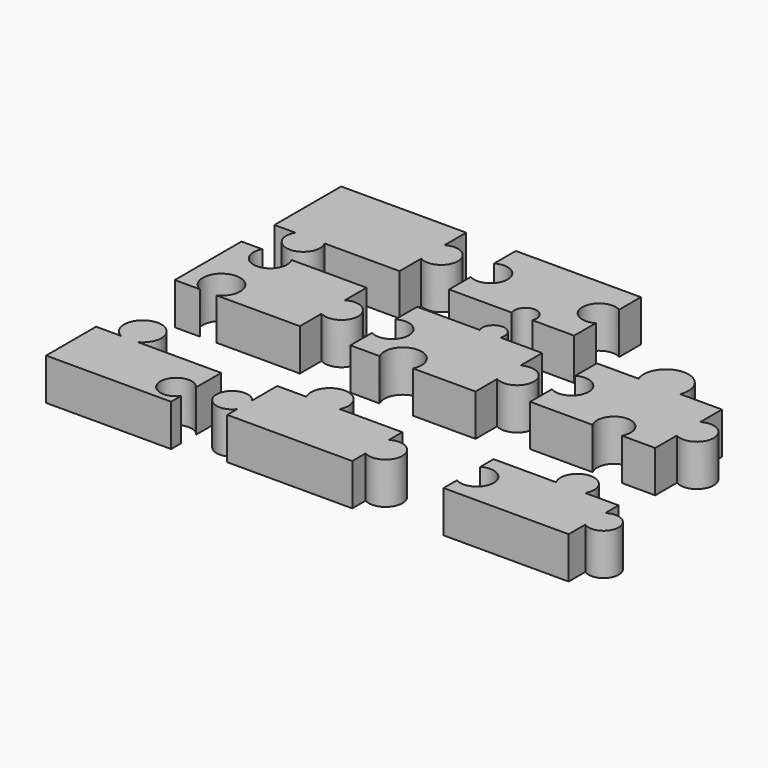
from build123d import *

# Parameters (mm, degrees)
F1_DEPTH  = 25.4
F3_DEPTH  = 25.4
F5_DEPTH  = 25.4
F7_DEPTH  = 25.4
F8_DEPTH  = 25.4
F10_DEPTH = 25.4
F12_DEPTH = 25.4
F14_DEPTH = 25.4
F16_DEPTH = 25.4


# Not quite as in the source:
# - a feature names something its author has since deleted; it is built from what else it names


with BuildPart() as f1:
    # F0 (on Top) → F1 (new body)
    with BuildSketch(Plane.XY):
        with BuildLine():
            Line((0, 16.51), (0, 0))
            Line((0, 0), (38.1, 0))
            ThreePointArc((38.1, 0), (44.45, 9.3791593051), (50.8, 0))
            Line((50.8, 0), (76.2, 0))
            Line((76.2, 0), (76.2, 16.51))
            ThreePointArc((76.2, 16.51), (60.8809326597, 25.4), (76.2, 34.29))
            Line((76.2, 34.29), (76.2, 50.8))
            Line((76.2, 50.8), (0, 50.8))
            Line((0, 50.8), (0, 34.29))
            ThreePointArc((0, 34.29), (15.3190673403, 25.4), (0, 16.51))
        make_face()
    extrude(amount=F1_DEPTH)


with BuildPart() as f3:
    # F2 (on Top) → F3 (new body)
    with BuildSketch(Plane.XY):
        Polygon((-30.1954353519, 34.29), (-30.1954353519, 50.8), (-106.3954353519, 50.8), (-106.3954353519, 0), (-93.6954353519, 0), (-75.9154353519, 0), (-30.1954353519, 0), (-30.1954353519, 16.51), align=None)
        with BuildLine():
            ThreePointArc((-30.1954353519, 16.51), (-14.8763680116, 25.4), (-30.1954353519, 34.29))
            Line((-30.1954353519, 34.29), (-30.1954353519, 16.51))
        make_face()
        with BuildLine():
            Line((-75.9154353519, 0), (-93.6954353519, 0))
            ThreePointArc((-93.6954353519, 0), (-84.8054353519, -15.3190673403), (-75.9154353519, 0))
        make_face()
    extrude(amount=F3_DEPTH)


with BuildPart() as f5:
    # F4 (on Top) → F5 (new body)
    with BuildSketch(Plane.XY):
        with BuildLine():
            Line((-31.7811166644, -39.6367072773), (-31.7811166644, -23.1267072773))
            Line((-31.7811166644, -23.1267072773), (-77.5011166644, -23.1267072773))
            ThreePointArc((-77.5011166644, -23.1267072773), (-86.3911166644, -38.4457746176), (-95.2811166644, -23.1267072773))
            Line((-95.2811166644, -23.1267072773), (-107.9811166644, -23.1267072773))
            Line((-107.9811166644, -23.1267072773), (-107.9811166644, -73.9267072773))
            Line((-107.9811166644, -73.9267072773), (-92.7411166644, -73.9267072773))
            ThreePointArc((-92.7411166644, -73.9267072773), (-87.6611166644, -52.4074819516), (-82.5811166644, -73.9267072773))
            Line((-82.5811166644, -73.9267072773), (-31.7811166644, -73.9267072773))
            Line((-31.7811166644, -73.9267072773), (-31.7811166644, -57.4167072773))
            Line((-31.7811166644, -57.4167072773), (-31.7811166644, -39.6367072773))
        make_face()
        with BuildLine():
            ThreePointArc((-31.7811166644, -57.4167072773), (-16.4620493241, -48.5267072773), (-31.7811166644, -39.6367072773))
            Line((-31.7811166644, -39.6367072773), (-31.7811166644, -57.4167072773))
        make_face()
    extrude(amount=F5_DEPTH)


with BuildPart() as f7:
    # F6 (on Top) → F7 (new body)
    with BuildSketch(Plane.XY):
        with BuildLine():
            ThreePointArc((50.1078782513, -23.4696016228), (43.7578782513, -14.0904423178), (37.4078782513, -23.4696016228))
            Line((37.4078782513, -23.4696016228), (50.1078782513, -23.4696016228))
        make_face()
        with BuildLine():
            ThreePointArc((75.5078782513, -57.7596016228), (90.8269455917, -48.8696016228), (75.5078782513, -39.9796016228))
            Line((75.5078782513, -39.9796016228), (75.5078782513, -57.7596016228))
        make_face()
        with BuildLine():
            Line((37.4078782513, -23.4696016228), (-0.6921217487, -23.4696016228))
            Line((-0.6921217487, -23.4696016228), (-0.6921217487, -39.9796016228))
            ThreePointArc((-0.6921217487, -39.9796016228), (14.6269455917, -48.8696016228), (-0.6921217487, -57.7596016228))
            Line((-0.6921217487, -57.7596016228), (-0.6921217487, -74.2696016228))
            Line((-0.6921217487, -74.2696016228), (17.0878782513, -74.2696016228))
            ThreePointArc((17.0878782513, -74.2696016228), (27.2478782513, -57.8303762971), (37.4078782513, -74.2696016228))
            Line((37.4078782513, -74.2696016228), (75.5078782513, -74.2696016228))
            Line((75.5078782513, -74.2696016228), (75.5078782513, -57.7596016228))
            Line((75.5078782513, -57.7596016228), (75.5078782513, -39.9796016228))
            Line((75.5078782513, -39.9796016228), (75.5078782513, -23.4696016228))
            Line((75.5078782513, -23.4696016228), (50.1078782513, -23.4696016228))
            Line((50.1078782513, -23.4696016228), (37.4078782513, -23.4696016228))
        make_face()
    extrude(amount=F7_DEPTH)


with BuildPart() as f8:
    # F0 (on Top) → F8 (new body)
    with BuildSketch(Plane.XY):
        with BuildLine():
            Line((0, 16.51), (0, 0))
            Line((0, 0), (38.1, 0))
            ThreePointArc((38.1, 0), (44.45, 9.3791593051), (50.8, 0))
            Line((50.8, 0), (76.2, 0))
            Line((76.2, 0), (76.2, 16.51))
            ThreePointArc((76.2, 16.51), (60.8809326597, 25.4), (76.2, 34.29))
            Line((76.2, 34.29), (76.2, 50.8))
            Line((76.2, 50.8), (0, 50.8))
            Line((0, 50.8), (0, 34.29))
            ThreePointArc((0, 34.29), (15.3190673403, 25.4), (0, 16.51))
        make_face()
    extrude(amount=F8_DEPTH)


with BuildPart() as f10:
    # F9 (on Top) → F10 (new body)
    with BuildSketch(Plane.XY):
        with BuildLine():
            ThreePointArc((153.2303552747, -15.5059827256), (140.5303552747, 3.2523358845), (127.8303552747, -15.5059827256))
            Line((127.8303552747, -15.5059827256), (153.2303552747, -15.5059827256))
        make_face()
        with BuildLine():
            ThreePointArc((178.6303552747, -49.7959827256), (193.949422615, -40.9059827256), (178.6303552747, -32.0159827256))
            Line((178.6303552747, -32.0159827256), (178.6303552747, -49.7959827256))
        make_face()
        with BuildLine():
            Line((127.8303552747, -15.5059827256), (102.4303552747, -15.5059827256))
            Line((102.4303552747, -15.5059827256), (102.4303552747, -32.0159827256))
            ThreePointArc((102.4303552747, -32.0159827256), (117.749422615, -40.9059827256), (102.4303552747, -49.7959827256))
            Line((102.4303552747, -49.7959827256), (102.4303552747, -66.3059827256))
            Line((102.4303552747, -66.3059827256), (140.5303552747, -66.3059827256))
            ThreePointArc((140.5303552747, -66.3059827256), (149.4203552747, -50.9869153853), (158.3103552747, -66.3059827256))
            Line((158.3103552747, -66.3059827256), (178.6303552747, -66.3059827256))
            Line((178.6303552747, -66.3059827256), (178.6303552747, -49.7959827256))
            Line((178.6303552747, -49.7959827256), (178.6303552747, -32.0159827256))
            Line((178.6303552747, -32.0159827256), (178.6303552747, -15.5059827256))
            Line((178.6303552747, -15.5059827256), (153.2303552747, -15.5059827256))
            Line((153.2303552747, -15.5059827256), (127.8303552747, -15.5059827256))
        make_face()
    extrude(amount=F10_DEPTH)


with BuildPart() as f12:
    # F11 (on Top) → F12 (new body)
    with BuildSketch(Plane.XY):
        with BuildLine():
            ThreePointArc((-81.7762166262, -134.8588719903), (-86.8562166262, -113.3396466646), (-91.9362166262, -134.8588719903))
            Line((-91.9362166262, -134.8588719903), (-81.7762166262, -134.8588719903))
        make_face()
        with BuildLine():
            Line((-91.9362166262, -134.8588719903), (-107.1762166262, -134.8588719903))
            Line((-107.1762166262, -134.8588719903), (-107.1762166262, -172.9588719903))
            Line((-107.1762166262, -172.9588719903), (-30.9762166262, -172.9588719903))
            Line((-30.9762166262, -172.9588719903), (-30.9762166262, -165.3388719903))
            ThreePointArc((-30.9762166262, -165.3388719903), (-48.1212166262, -159.6238719903), (-30.9762166262, -153.9088719903))
            Line((-30.9762166262, -153.9088719903), (-30.9762166262, -134.8588719903))
            Line((-30.9762166262, -134.8588719903), (-81.7762166262, -134.8588719903))
            Line((-81.7762166262, -134.8588719903), (-91.9362166262, -134.8588719903))
        make_face()
    extrude(amount=F12_DEPTH)


with BuildPart() as f14:
    # F13 (on Top) → F14 (new body)
    with BuildSketch(Plane.XY):
        Polygon((16.0720860608, -128.7438145399), (-1.7079139392, -128.7438145399), (-1.7079139392, -147.7938145399), (-1.7079139392, -159.2238145399), (-1.7079139392, -166.8438145399), (74.4920860608, -166.8438145399), (74.4920860608, -156.6838145399), (74.4920860608, -138.9038145399), (74.4920860608, -128.7438145399), (36.3920860608, -128.7438145399), align=None)
        with BuildLine():
            ThreePointArc((36.3920860608, -128.7438145399), (26.2320860608, -112.3045892142), (16.0720860608, -128.7438145399))
            Line((16.0720860608, -128.7438145399), (36.3920860608, -128.7438145399))
        make_face()
        with BuildLine():
            Line((-1.7079139392, -159.2238145399), (-1.7079139392, -147.7938145399))
            ThreePointArc((-1.7079139392, -147.7938145399), (-18.8529139392, -153.5088145399), (-1.7079139392, -159.2238145399))
        make_face()
        with BuildLine():
            ThreePointArc((74.4920860608, -156.6838145399), (89.8111534011, -147.7938145399), (74.4920860608, -138.9038145399))
            Line((74.4920860608, -138.9038145399), (74.4920860608, -156.6838145399))
        make_face()
    extrude(amount=F14_DEPTH)


with BuildPart() as f16:
    # F15 (on Top) → F16 (new body)
    with BuildSketch(Plane.XY):
        with BuildLine():
            ThreePointArc((181.6284889733, -123.3046403503), (172.7384889733, -107.98557301), (163.8484889733, -123.3046403503))
            Line((163.8484889733, -123.3046403503), (181.6284889733, -123.3046403503))
        make_face()
        with BuildLine():
            Line((163.8484889733, -123.3046403503), (125.7484889733, -123.3046403503))
            Line((125.7484889733, -123.3046403503), (125.7484889733, -133.4646403503))
            ThreePointArc((125.7484889733, -133.4646403503), (141.0675563136, -142.3546403503), (125.7484889733, -151.2446403503))
            Line((125.7484889733, -151.2446403503), (125.7484889733, -161.4046403503))
            Line((125.7484889733, -161.4046403503), (201.9484889733, -161.4046403503))
            Line((201.9484889733, -161.4046403503), (201.9484889733, -148.7046403503))
            Line((201.9484889733, -148.7046403503), (201.9484889733, -133.4646403503))
            Line((201.9484889733, -133.4646403503), (201.9484889733, -123.3046403503))
            Line((201.9484889733, -123.3046403503), (181.6284889733, -123.3046403503))
            Line((181.6284889733, -123.3046403503), (163.8484889733, -123.3046403503))
        make_face()
        with BuildLine():
            ThreePointArc((201.9484889733, -148.7046403503), (216.186589213, -141.0846403503), (201.9484889733, -133.4646403503))
            Line((201.9484889733, -133.4646403503), (201.9484889733, -148.7046403503))
        make_face()
    extrude(amount=F16_DEPTH)


solid = Compound([f1.part, f3.part, f5.part, f7.part, f8.part, f10.part, f12.part, f14.part, f16.part])
